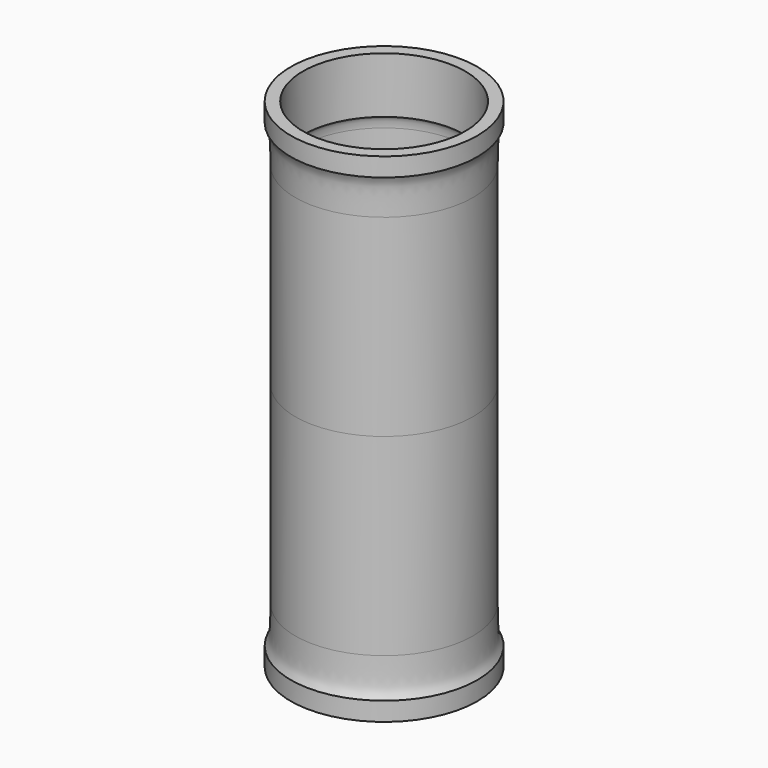
from build123d import *


with BuildPart() as f1:
    # F0 (on Front) → F1 (revolve)
    with BuildSketch(Plane.XZ):
        with BuildLine():
            Line((25, 66.7063602807), (21.75, 66.7063602807))
            Line((21.75, 66.7063602807), (21.75, 51.7063602807))
            add(Edge.make_bspline(
                [(21.75, 51.7063602807), (22.356479466, 51.0745504571), (22.5, 49.8551437309), (22.5, 48.7063602807)],
                knots=[0, 0, 0, 0, 3.0923292192, 3.0923292192, 3.0923292192, 3.0923292192], degree=3))
            Line((22.5, 48.7063602807), (22.5, 0))
            Line((22.5, 0), (23.8, 0))
            Line((23.8, 0), (23.8, 51.7063602807))
            add(Edge.make_bspline(
                [(25, 61.7063602807), (23.8398276269, 59.9064195158), (23.8, 58.3514220487), (23.8, 51.7063602807)],
                knots=[0, 0, 0, 0, 10.0717426496, 10.0717426496, 10.0717426496, 10.0717426496], degree=3))
            Line((25, 61.7063602807), (25, 66.7063602807))
        make_face()
    revolve(axis=Axis((0, 0, 33.3531801404), (0, 0, -1)))

    # F2: F1 across face


with BuildPart() as f1_1:
    add(f1.part)
    add(f1.part.mirror(Plane(origin=(0, 0, 0), x_dir=(1, 0, 0), z_dir=(0, 0, -1))))


solid = f1_1.part
